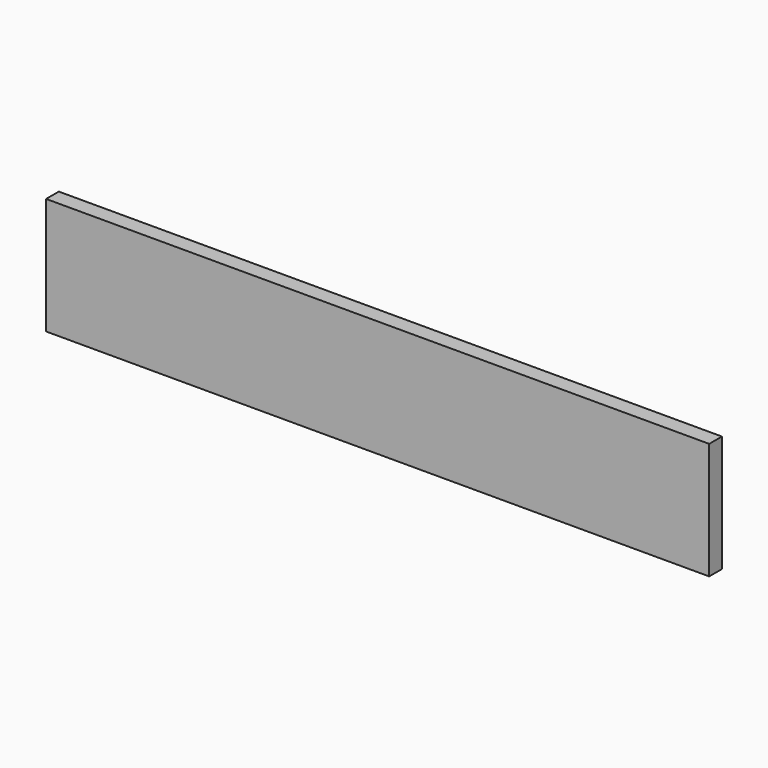
from build123d import *

# Parameters (mm, degrees)
F0_W      = 500
F0_H      = 500
F1_DEPTH  = 12
F2_W      = 500
F2_H      = 50
F3_DEPTH  = 6
F6_DEPTH  = 6
F14_DEPTH = 6
F15_R     = 19.99999
F19_DEPTH = 6
F22_DEPTH = 12
F25_DEPTH = 6
F27_W     = 12
F27_H     = 320
F28_DEPTH = 44
F31_W     = 196
F31_H     = 12
F32_DEPTH = 44
F37_DEPTH = 3
F43_DEPTH = 12


# Not quite as in the source:
# - a fillet or chamfer is up to 0.001 mm smaller than in the source, because OpenCascade refuses the exact size


with BuildPart() as f1:
    # F0 (on Top) → F1 (new body)
    with BuildSketch(Plane.XY):
        Rectangle(F0_W, F0_H)
    extrude(amount=F1_DEPTH)


with BuildPart() as f3:
    # F2 (on Right) → F3 (new body, symmetric)
    with BuildSketch(Plane.YZ):
        Rectangle(F2_W, F2_H)
    extrude(amount=F3_DEPTH, both=True)


with BuildPart() as f3_1:
    # F4: moved
    add(f3.part.moved(Location((0, 0, -25))))


with BuildPart() as f6:
    # F5 (on Front) → F6 (new body, symmetric)
    with BuildSketch(Plane.XZ):
        Polygon((-250, -25), (250, -25), (250, 25), (6, 25), (6, 0), (-6, 0), (-6, 25), (-250, 25), align=None)
    extrude(amount=F6_DEPTH, both=True)


with BuildPart() as f6_1:
    # F7: moved
    add(f6.part.moved(Location((0, 80, -25))))


with BuildPart() as f8_1:
    # F8: copy of F6
    add(f6_1.part)


with BuildPart() as f3_2:
    add(f3_1.part)

    # F10: cut F6
    add(f6_1.part, mode=Mode.SUBTRACT)


with BuildPart() as f11_1:
    # F11: copy of F6
    add(f6_1.part.moved(Location((0, 164, 0))))


with BuildPart() as f3_3:
    add(f3_2.part)

    # F12: cut F11_1
    add(f11_1.part, mode=Mode.SUBTRACT)


with BuildPart() as f14:
    # F13 (on Right) → F14 (new body, symmetric)
    with BuildSketch(Plane.YZ):
        Polygon((250, -50), (250, 0), (250, 452), (70, 452), (-110, 452), (-250, 100), (-250, -50), align=None)
        Polygon((0, 412), (70, 412), (140, 412), (140, 372), (0, 372), align=None, mode=Mode.SUBTRACT)
    extrude(amount=F14_DEPTH, both=True)

    # F15 (radius 20 in the source; OpenCascade refuses exactly that, so slightly less here)
    f15_edges = [f14.edges().sort_by_distance(p)[0] for p in [
        (0, 140, 372),
        (0, 140, 412),
        (0, 0, 412),
        (0, 0, 372),
    ]]
    fillet(f15_edges, radius=F15_R)


with BuildPart() as f14_1:
    # F16: moved
    add(f14.part.moved(Location((-256, 0, 0))))


with BuildPart() as f17_1:
    # F17: copy of F14
    add(f14_1.part.moved(Location((512, 0, 0))))


with BuildPart() as f19:
    # F18 (on Front) → F19 (new body, symmetric)
    with BuildSketch(Plane.XZ):
        Polygon((-262, 452), (-262, 0), (-262, -50), (262, -50), (262, 452), align=None)
    extrude(amount=F19_DEPTH, both=True)


with BuildPart() as f19_1:
    # F20: moved
    add(f19.part.moved(Location((0, 256, 0))))


with BuildPart() as f22:
    # F21 (on face) → F22 (new body)
    with BuildSketch(Plane.XY.offset(12)):
        Polygon((262, 262), (0, 262), (-262, 262), (-262, -110), (262, -110), align=None)
    extrude(amount=F22_DEPTH)


with BuildPart() as f22_1:
    # F23: moved
    add(f22.part.moved(Location((0, 0, 440))))


with BuildPart() as f25:
    # F24 (on Front) → F25 (new body, symmetric)
    with BuildSketch(Plane.XZ):
        Polygon((-250, 12), (0, 12), (250, 12), (250, 100), (-250, 100), align=None)
    extrude(amount=F25_DEPTH, both=True)


with BuildPart() as f25_1:
    # F26: moved
    add(f25.part.moved(Location((0, -244, 0))))


with BuildPart() as f28:
    # F27 (on Top) → F28 (new body)
    with BuildSketch(Plane.XY):
        with Locations((-24, -90)):
            Rectangle(F27_W, F27_H)
    extrude(amount=F28_DEPTH)


with BuildPart() as f28_1:
    # F29: moved
    add(f28.part.moved(Location((0, 0, -48))))


with BuildPart() as f30_1:
    # F30: copy of F28
    add(f28_1.part.moved(Location((-208, 0, 0))))


with BuildPart() as f32:
    # F31 (on Top) → F32 (new body)
    with BuildSketch(Plane.XY):
        with Locations((-128, -244)):
            Rectangle(F31_W, F31_H)
    extrude(amount=-F32_DEPTH)


with BuildPart() as f32_1:
    # F33: moved
    add(f32.part.moved(Location((0, 0, -4))))


with BuildPart() as f34_1:
    # F34: copy of F32
    add(f32_1.part.moved(Location((0, 308, 0))))


with BuildPart() as f35_1:
    # F35: copy of F32
    add(f32_1.part.moved(Location((256, 0, 0))))


with BuildPart() as f35_2:
    # F35: copy of F30_1
    add(f30_1.part.moved(Location((256, 0, 0))))


with BuildPart() as f35_3:
    # F35: copy of F28
    add(f28_1.part.moved(Location((256, 0, 0))))


with BuildPart() as f35_4:
    # F35: copy of F34_1
    add(f34_1.part.moved(Location((256, 0, 0))))


with BuildPart() as f37:
    # F36 (on Top) → F37 (new body)
    with BuildSketch(Plane.XY):
        Polygon((-24, -244), (-24, 0), (-24, 64), (-232, 64), (-232, -244), align=None)
    extrude(amount=F37_DEPTH)


with BuildPart() as f37_1:
    # F38: moved
    add(f37.part.moved(Location((0, 0, -44))))


with BuildPart() as f39_1:
    # F39: copy of F37
    add(f37_1.part.moved(Location((256, 0, 0))))


with BuildPart() as f30_1_1:
    add(f30_1.part)

    # F40: cut F37
    add(f37_1.part, mode=Mode.SUBTRACT)


with BuildPart() as f32_2:
    add(f32_1.part)

    # F40: cut F37
    add(f37_1.part, mode=Mode.SUBTRACT)


with BuildPart() as f28_2:
    add(f28_1.part)

    # F40: cut F37
    add(f37_1.part, mode=Mode.SUBTRACT)


with BuildPart() as f34_1_1:
    add(f34_1.part)

    # F40: cut F37
    add(f37_1.part, mode=Mode.SUBTRACT)


with BuildPart() as f35_1_1:
    add(f35_1.part)

    # F41: cut F39_1
    add(f39_1.part, mode=Mode.SUBTRACT)


with BuildPart() as f35_3_1:
    add(f35_3.part)

    # F41: cut F39_1
    add(f39_1.part, mode=Mode.SUBTRACT)


with BuildPart() as f35_4_1:
    add(f35_4.part)

    # F41: cut F39_1
    add(f39_1.part, mode=Mode.SUBTRACT)


with BuildPart() as f35_2_1:
    add(f35_2.part)

    # F41: cut F39_1
    add(f39_1.part, mode=Mode.SUBTRACT)


with BuildPart() as f43:
    # F42 (on Front) → F43 (new body)
    with BuildSketch(Plane.XZ):
        Polygon((0, 12), (0, 0), (0, -50), (262, -50), (262, 12), align=None)
    extrude(amount=F43_DEPTH)


with BuildPart() as f43_1:
    # F44: moved
    add(f43.part.moved(Location((0, -250, 0))))


with BuildPart() as f45_1:
    # F45: copy of F43
    add(f43_1.part.moved(Location((-262, 0, 0))))


solid = f25_1.part
